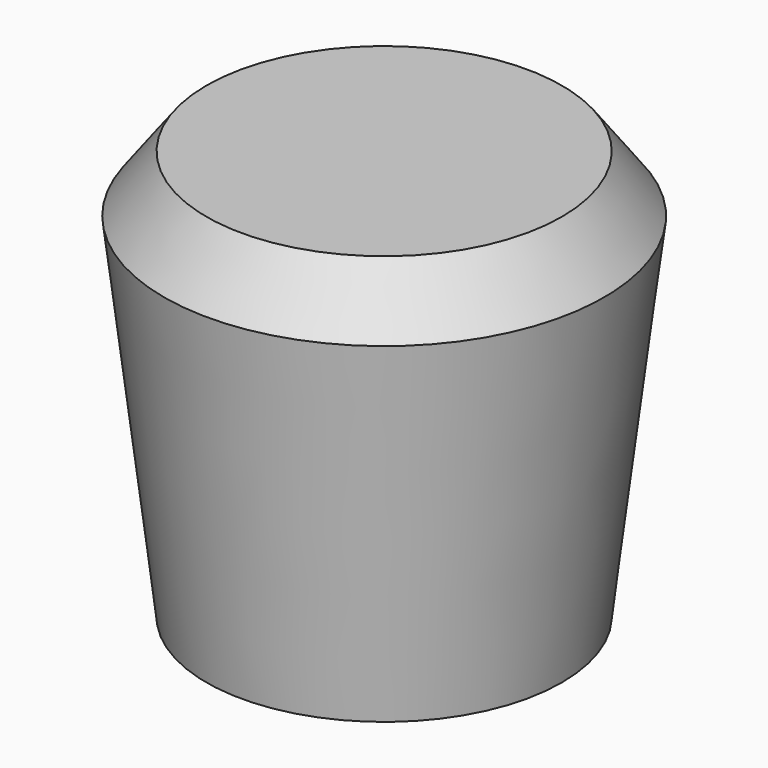
from build123d import *

# Parameters (mm, degrees)
F2_R     = 9.652
F3_DEPTH = 33.02


# Not quite as in the source:
# - a feature names something its author has since deleted; it is built from what else it names


with BuildPart() as f1:
    # F0 (on Front) → F1 (revolve)
    with BuildSketch(Plane.XZ):
        Polygon((-70.1680659715, 31.024657777), (-65.6206389772, -6.8029896218), (-46.5706389772, -6.8029896218), (-46.5706389772, 37.1390103782), (-65.6206389772, 37.1390103782), align=None)
    revolve(axis=Axis((-46.5706389772, 0, 15.1680103782), (0, 0, -1)))

    # F2 (on face) → F3 (cut)
    with BuildSketch(Plane(origin=(0, 0, -6.8029896218), x_dir=(1, 0, 0), z_dir=(0, 0, -1))):
        with Locations((-46.5706389772, 0)):
            Circle(F2_R)
    extrude(amount=-F3_DEPTH, mode=Mode.SUBTRACT)


solid = f1.part
